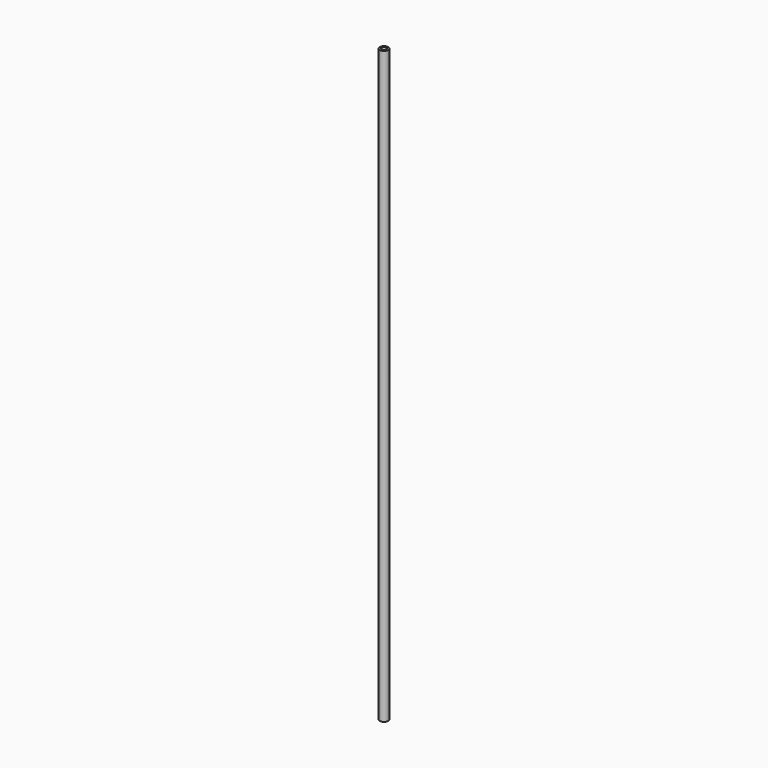
from build123d import *

# Parameters (mm, degrees)
F1_R     = 10.715625
F1_R_2   = 6.35
F2_DEPTH = 1524


# Not quite as in the source:
# - a variable given as a bare number and used for a length is read in inches; the dataset says mm whatever the document's units were


with BuildPart() as f2:
    # F1 (on Top) → F2 (new body)
    with BuildSketch(Plane.XY):
        Circle(F1_R)
        Circle(F1_R_2, mode=Mode.SUBTRACT)
    extrude(amount=F2_DEPTH)


solid = f2.part
